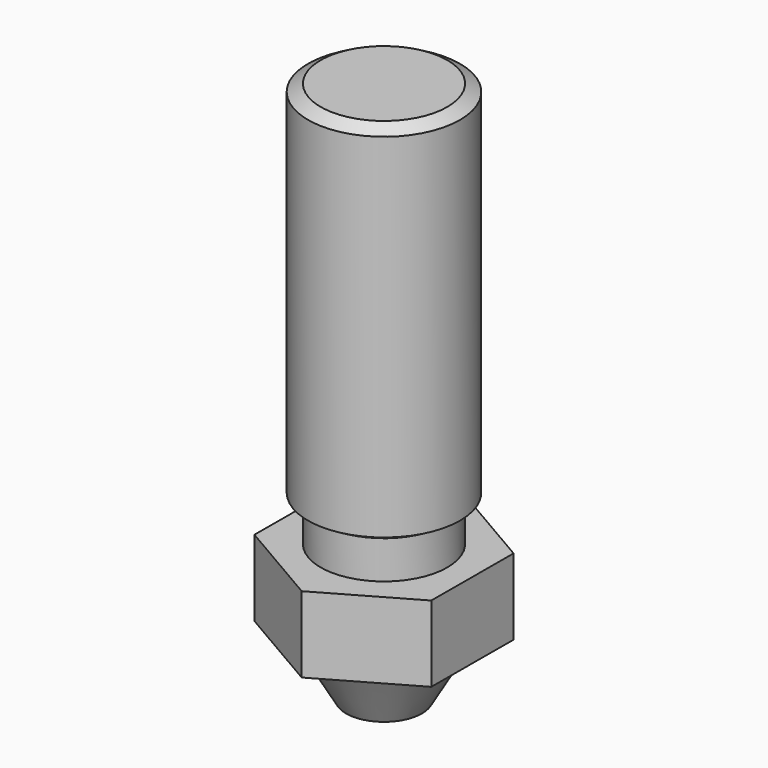
from build123d import *

# Parameters (mm, degrees)
F3_DEPTH   = 3
F4_R       = 2.5
F5_DEPTH   = 1.5
F6_R       = 3
F7_DEPTH   = 14.5
F8_SIZE2   = 0.2886751346
F8_SIZE    = 0.5
F8_2_SIZE2 = 0.288665
F8_2_SIZE  = 0.49999


# Not quite as in the source:
# - a fillet or chamfer is up to 0.001 mm smaller than in the source, because OpenCascade refuses the exact size


with BuildPart() as f1:
    # F0 (on Front) → F1 (revolve)
    with BuildSketch(Plane.XZ):
        Polygon((0, 2.4), (0, 0), (0.9, 0), (2.2856406461, 2.4), align=None)
    revolve(axis=Axis((-0.6, 0, 1.2), (0, 0, 1)))

    # F2 (on face) → F3 (join)
    with BuildSketch(Plane.XY.offset(2.4)):
        Polygon((2.9073034694, 2.0080228353), (-0.5853470521, 4.0414253209), (-4.0926505214, 2.0334024856), (-4.1073034694, -2.0080228353), (-0.6146529479, -4.0414253209), (2.8926505214, -2.0334024856), align=None)
    extrude(amount=F3_DEPTH)

    # F4 (on face) → F5 (join)
    with BuildSketch(Plane.XY.offset(5.4)):
        with Locations((-0.6, 0)):
            Circle(F4_R)
    extrude(amount=F5_DEPTH)

    # F6 (on face) → F7 (join)
    with BuildSketch(Plane.XY.offset(6.9)):
        with Locations((-0.6, 0)):
            Circle(F6_R)
    extrude(amount=F7_DEPTH)

    # F8
    f8_edges = [f1.edges().sort_by_distance(p)[0] for p in [
        (-3.6, 0, 21.4),
    ]]
    f8_side = f1.faces().sort_by_distance((-0.6, 0, 21.4))[0]
    chamfer(f8_edges, length=F8_SIZE, length2=F8_SIZE2, reference=f8_side)

    # F8#2 (size 0.5 and 0.2886751346 in the source; OpenCascade refuses exactly that, so slightly less here)
    f8_2_edges = [f1.edges().sort_by_distance(p)[0] for p in [
        (-3.6, 0, 6.9),
    ]]
    f8_2_side = f1.faces().sort_by_distance((-3.515147, 0, 6.9))[0]
    chamfer(f8_2_edges, length=F8_2_SIZE, length2=F8_2_SIZE2, reference=f8_2_side)


solid = f1.part
